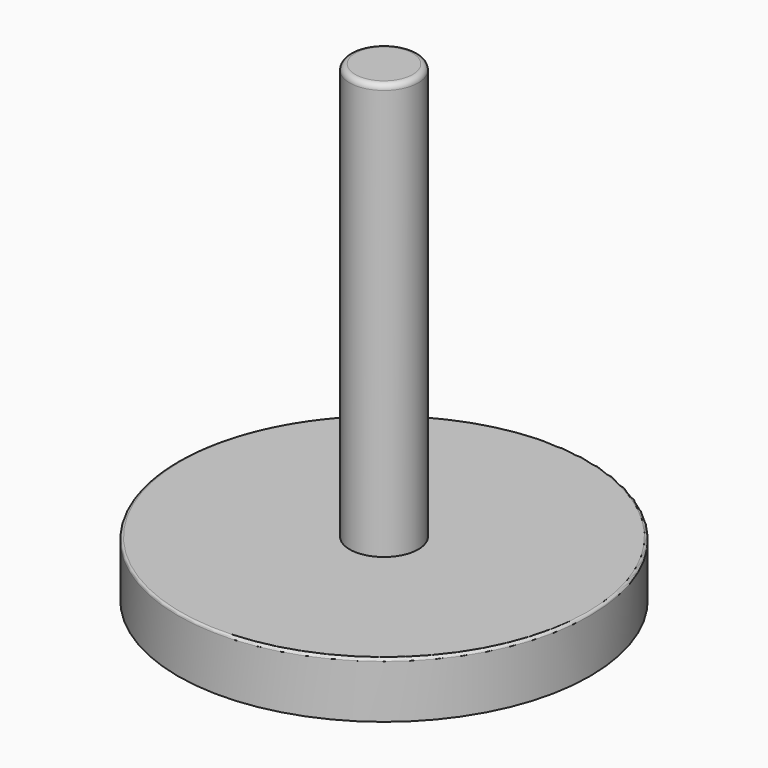
from build123d import *

# Parameters (mm, degrees)
F2_W            = 17
F2_H            = 4
F3_DEPTH        = 12
F3_COPIES_COUNT = 6
F4_R            = 0.59
F5_R            = 1.3


# Not quite as in the source:
# - a pattern or mirror of a feature is missing from the dataset's text; its kind, count and spacing are read off the source's solid


with BuildPart() as f1:
    # F0 (on Front) → F1 (revolve)
    with BuildSketch(Plane.XZ):
        Polygon((0, 110), (0, 40), (9, 0), (48, 0), (48, 13), (8, 13), (8, 110), align=None)
    revolve(axis=Axis((0, 0, 75), (0, 0, 1)))

    # F2 (on face) → F3 (cut)
    with BuildSketch(Plane(origin=(0, 0, 0), x_dir=(1, 0, 0), z_dir=(0, 0, -1))):
        with Locations((0, 43)):
            Rectangle(F2_W, F2_H)
    f3 = extrude(amount=-F3_DEPTH, mode=Mode.SUBTRACT)

    # F3_copies: F3 ×6 about axis
    f3_copies_axis = Axis((0, 0, 0), (0, 0, 1))
    for i in range(1, F3_COPIES_COUNT):
        add(f3.rotate(f3_copies_axis, i * 360 / F3_COPIES_COUNT), mode=Mode.SUBTRACT)

    # F4
    f4_edges = [f1.edges().sort_by_distance(p)[0] for p in [
        (-48, 0, 13),
    ]]
    fillet(f4_edges, radius=F4_R)

    # F5
    f5_edges = [f1.edges().sort_by_distance(p)[0] for p in [
        (-8, 0, 110),
    ]]
    fillet(f5_edges, radius=F5_R)


solid = f1.part
